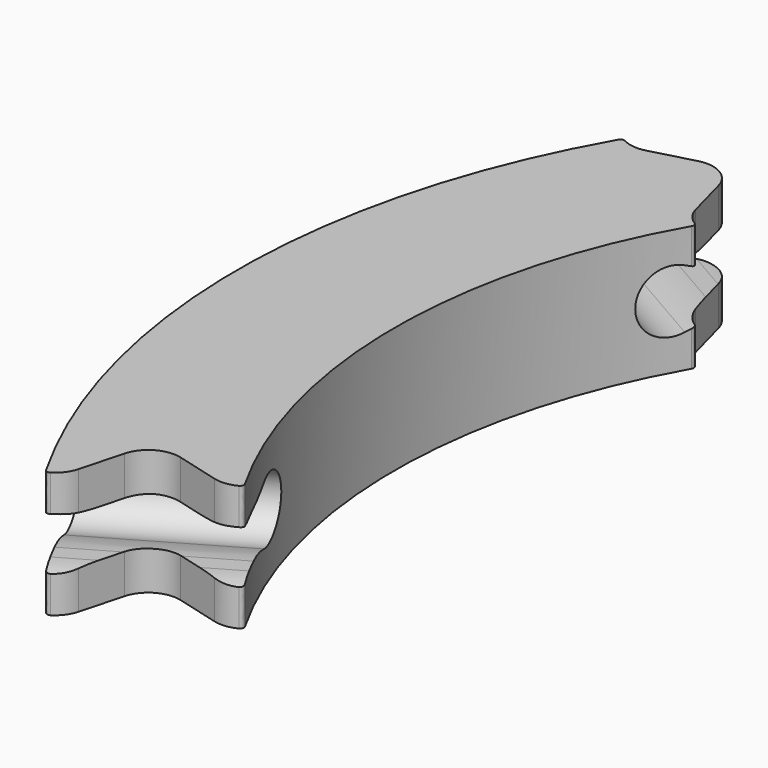
from build123d import *

# Parameters (mm, degrees)
F0_W          = 254
F0_H          = 203.2
F1_ANGLE_BACK = 30
F1_ANGLE      = 60
F3_DEPTH      = 203.2
F5_DEPTH      = 203.2
F9_DEPTH      = 254
F11_DEPTH     = 254
F13_DEPTH     = 76.2
F14_R         = 50.8
F15_R         = 50.8
F16_R         = 6.35


with BuildPart() as f1:
    # F0 (on Front) → F1 (revolve)
    with BuildSketch(Plane.XZ, mode=Mode.PRIVATE) as f1_sk:
        with Locations((-1041.4, 0)):
            Rectangle(F0_W, F0_H)
    revolve(f1_sk.sketch.rotate(Axis((0, 0, 0), (0, 0, -1)), -F1_ANGLE_BACK), axis=Axis((0, 0, 0), (0, 0, -1)), revolution_arc=F1_ANGLE)

    # F2 (on face) → F3 (join, through all)
    with BuildSketch(Plane.XY.offset(101.6)):
        Polygon((-851.0788555011, 608.6881810245), (-989.8670365256, 571.5), (-813.8906744766, 469.9), align=None)
    extrude(amount=-F3_DEPTH)

    # F4 (on face) → F5 (cut, through all)
    with BuildSketch(Plane.XY.offset(101.6)):
        Polygon((-952.6788555011, -432.7118189755), (-989.8670365256, -571.5), (-813.8906744766, -469.9), align=None)
    extrude(amount=-F5_DEPTH, mode=Mode.SUBTRACT)

    # F8 (on face) → F9 (cut, symmetric)
    with BuildSketch(Plane(origin=(-901.8788555011, 520.7, 0), x_dir=(0.5, 0.8660254038, 0), z_dir=(0.8660254038, -0.5, 0))):
        with BuildLine():
            ThreePointArc((37.1095657574, 38.1), (10.1687973942, 40.50015), (-15.9233897985, 47.625))
            ThreePointArc((-15.9233897985, 47.625), (-84.4010416505, 0), (-15.9233897985, -47.625))
            ThreePointArc((-15.9233897985, -47.625), (10.1687973942, -40.50015), (37.1095657574, -38.1))
            Line((37.1095657574, -38.1), (64.4904342426, -38.1))
            ThreePointArc((64.4904342426, -38.1), (91.4312026058, -40.50015), (117.5233897985, -47.625))
            ThreePointArc((117.5233897985, -47.625), (186.0010416505, 0), (117.5233897985, 47.625))
            ThreePointArc((117.5233897985, 47.625), (91.4312026058, 40.50015), (64.4904342426, 38.1))
            Line((64.4904342426, 38.1), (37.1095657574, 38.1))
        make_face()
    extrude(amount=F9_DEPTH, both=True, mode=Mode.SUBTRACT)

    # F10 (on face) → F11 (cut, symmetric)
    with BuildSketch(Plane(origin=(-901.8788555011, -520.7, 0), x_dir=(0.5, -0.8660254038, 0), z_dir=(-0.8660254038, -0.5, 0))):
        with BuildLine():
            ThreePointArc((-64.4904342426, 38.1), (-91.4312026058, 40.50015), (-117.5233897985, 47.625))
            ThreePointArc((-117.5233897985, 47.625), (-186.0010416505, 0), (-117.5233897985, -47.625))
            ThreePointArc((-117.5233897985, -47.625), (-91.4312026058, -40.50015), (-64.4904342426, -38.1))
            Line((-64.4904342426, -38.1), (-37.1095657574, -38.1))
            ThreePointArc((-37.1095657574, -38.1), (-10.1687973942, -40.50015), (15.9233897985, -47.625))
            ThreePointArc((15.9233897985, -47.625), (84.4010416505, 0), (15.9233897985, 47.625))
            ThreePointArc((15.9233897985, 47.625), (-10.1687973942, 40.50015), (-37.1095657574, 38.1))
            Line((-37.1095657574, 38.1), (-64.4904342426, 38.1))
        make_face()
    extrude(amount=F11_DEPTH, both=True, mode=Mode.SUBTRACT)

    # F12 (on face) → F13 (cut)
    with BuildSketch(Plane(origin=(0, 0, -101.6), x_dir=(1, 0, 0), z_dir=(0, 0, -1))):
        with BuildLine():
            ThreePointArc((-965.2, 25.4), (-972.6394877579, 43.3605122421), (-990.6, 50.8))
            Line((-990.6, 50.8), (-1092.2, 50.8))
            ThreePointArc((-1092.2, 50.8), (-1110.1605122421, 43.3605122421), (-1117.6, 25.4))
            Line((-1117.6, 25.4), (-1117.6, -25.4))
            ThreePointArc((-1117.6, -25.4), (-1110.1605122421, -43.3605122421), (-1092.2, -50.8))
            Line((-1092.2, -50.8), (-990.6, -50.8))
            ThreePointArc((-990.6, -50.8), (-972.6394877579, -43.3605122421), (-965.2, -25.4))
            Line((-965.2, -25.4), (-965.2, 25.4))
        make_face()
    extrude(amount=-F13_DEPTH, mode=Mode.SUBTRACT)

    # F14
    f14_edges = [f1.edges().sort_by_distance(p)[0] for p in [
        (-813.890674, -469.9, 72.143572),
        (-989.867037, -571.5, 72.143572),
        (-989.867037, -571.5, -72.143572),
        (-813.890674, -469.9, -72.143572),
        (-813.890674, 469.9, 72.143572),
        (-989.867037, 571.5, 72.143572),
        (-989.867037, 571.5, -72.143572),
        (-813.890674, 469.9, -72.143572),
    ]]
    fillet(f14_edges, radius=F14_R)

    # F15
    f15_edges = [f1.edges().sort_by_distance(p)[0] for p in [
        (-952.678856, -432.711819, 72.143572),
        (-952.678856, -432.711819, -72.143572),
        (-851.078856, 608.688181, 72.143572),
        (-851.078856, 608.688181, -72.143572),
    ]]
    fillet(f15_edges, radius=F15_R)

    # F16
    f16_edges = [f1.edges().sort_by_distance(p)[0] for p in [
        (-791.893629, -457.2, 72.143572),
        (-791.893629, -457.2, -72.143572),
        (-1011.864082, -584.2, 72.143572),
        (-1011.864082, -584.2, -72.143572),
        (-791.893629, 457.2, 72.143572),
        (-791.893629, 457.2, -72.143572),
        (-1011.864082, 584.2, 72.143572),
        (-1011.864082, 584.2, -72.143572),
    ]]
    fillet(f16_edges, radius=F16_R)


solid = f1.part
